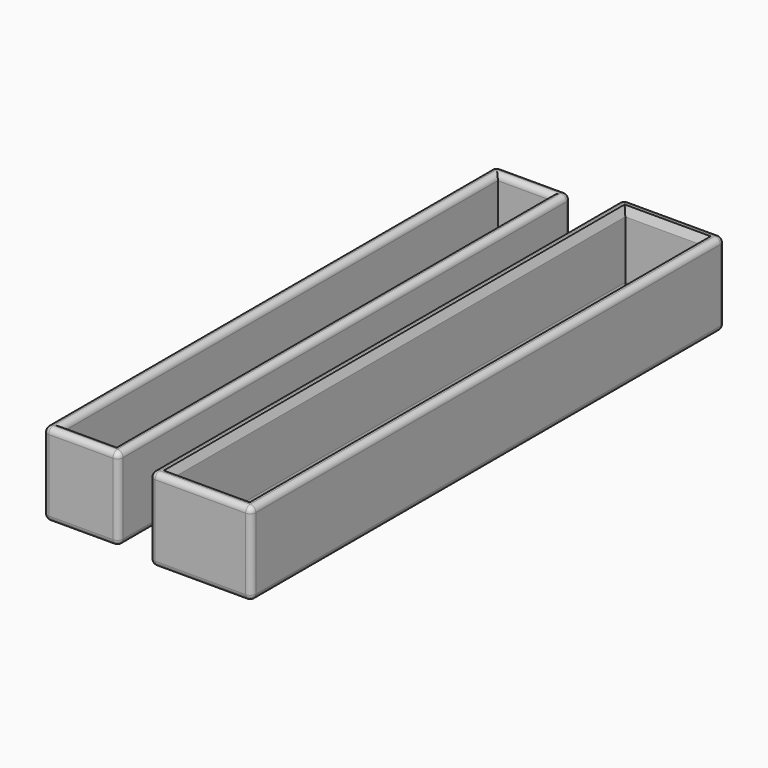
from build123d import *

# Parameters (mm, degrees)
F0_W          = 20
F0_H          = 150
F1_DEPTH      = 22
F2_T          = -3
F3_W          = 27
F3_H          = 157
F4_DEPTH      = 22
F5_T          = -3
F6_R          = 1.49999
F6_2_R        = 1.49999
F7_SIZE       = 0.9
F8_T4_DEPTH   = 21
F8_T9_DEPTH   = 24.3704715108
F8_T15_DEPTH  = 21
F8_T21_DEPTH  = 21
F8_T26_DEPTH  = 24.3704715108
F8_T32_DEPTH  = 151
F8_T37_DEPTH  = 154.3704715108
F8_T43_DEPTH  = 151
F8_T49_DEPTH  = 151
F8_T54_DEPTH  = 154.3704715108
F8_T60_DEPTH  = 151
F8_T65_DEPTH  = 154.3704715108
F8_T71_DEPTH  = 151
F8_T77_DEPTH  = 151
F8_T82_DEPTH  = 154.3704715108
F8_T88_DEPTH  = 21
F8_T93_DEPTH  = 24.3704715108
F8_T99_DEPTH  = 21
F8_T105_DEPTH = 21
F8_T110_DEPTH = 24.3704715108
F8_T117_DEPTH = 24.3704715108
F8_T122_DEPTH = 154.3704715108
F8_T130_DEPTH = 24.3704715108
F8_T135_DEPTH = 154.3704715108
F8_T143_DEPTH = 154.3704715108
F8_T148_DEPTH = 24.3704715108
F8_T156_DEPTH = 154.3704715108
F8_T161_DEPTH = 24.3704715108


# Not quite as in the source:
# - a fillet or chamfer that OpenCascade refuses, or shapes differently, is made with other operations: its cross-section is extruded or revolved along the edge and cut away or added
# - a fillet or chamfer is up to 0.001 mm smaller than in the source, because OpenCascade refuses the exact size


with BuildPart() as f1:
    # F0 (on Top) → F1 (new body)
    with BuildSketch(Plane.XY):
        with Locations((-29.877627335, 2.0745843649)):
            Rectangle(F0_W, F0_H)
    extrude(amount=F1_DEPTH)

    # F2
    f2_openings = [f1.faces().sort_by_distance(p)[0] for p in [
        (-29.877627, 2.074584, 22),
    ]]
    offset(amount=F2_T, openings=f2_openings)

    # F6 (radius 1.5 in the source; OpenCascade refuses exactly that, so slightly less here)
    f6_edges = [f1.edges().sort_by_distance(p)[0] for p in [
        (-19.877627, 2.074584, 22),
        (-22.877627, 2.074584, 22),
        (-29.877627, 77.074584, 22),
        (-29.877627, 74.074584, 22),
        (-39.877627, 2.074584, 22),
        (-36.877627, 2.074584, 22),
        (-29.877627, -69.925416, 22),
        (-29.877627, -72.925416, 22),
        (-39.877627, 2.074584, 0),
        (-39.877627, -72.925416, 11),
        (-29.877627, -72.925416, 0),
        (-19.877627, -72.925416, 11),
        (-19.877627, 77.074584, 11),
        (-39.877627, 77.074584, 11),
        (-29.877627, 77.074584, 0),
        (-19.877627, 2.074584, 0),
        (-36.877627, 2.074584, 3),
        (-29.877627, -69.925416, 3),
        (-29.877627, 74.074584, 3),
        (-22.877627, 2.074584, 3),
    ]]
    fillet(f6_edges, radius=F6_R)


with BuildPart() as f4:
    # F3 (on Top) → F4 (new body)
    with BuildSketch(Plane.XY):
        with Locations((3.5, 3.5)):
            Rectangle(F3_W, F3_H)
    extrude(amount=F4_DEPTH)

    # F5
    f5_openings = [f4.faces().sort_by_distance(p)[0] for p in [
        (3.5, 3.5, 22),
    ]]
    offset(amount=F5_T, openings=f5_openings)

    # F6#2 (radius 1.5 in the source; OpenCascade refuses exactly that, so slightly less here)
    f6_2_edges = [f4.edges().sort_by_distance(p)[0] for p in [
        (3.5, 82, 22),
        (-10, 3.5, 22),
        (17, 3.5, 22),
        (3.5, -75, 22),
        (3.5, -75, 0),
        (17, -75, 11),
        (17, 3.5, 0),
        (-10, 3.5, 0),
        (-10, -75, 11),
        (-10, 82, 11),
        (17, 82, 11),
        (3.5, 82, 0),
        (3.5, 79, 3),
        (14, 3.5, 3),
        (-7, 3.5, 3),
        (3.5, -72, 3),
    ]]
    fillet(f6_2_edges, radius=F6_2_R)

    # F7
    f7_edges = [f4.edges().sort_by_distance(p)[0] for p in [
        (3.5, 79, 22),
        (-7, 3.5, 22),
        (14, 3.5, 22),
        (3.5, -72, 22),
    ]]
    chamfer(f7_edges, length=F7_SIZE)

    # F8: chamfer of 1.3 on 4 edges, made by hand


with BuildPart() as f8_tool2:
    # F8_s3 → F8_t4 (new body)
    with BuildSketch(Plane.YZ.offset(14)):
        Polygon((79.9192388155, 22.0192388155), (79, 19.8), (79, 21.1), align=None)
    extrude(amount=-F8_T4_DEPTH)

    split(bisect_by=Plane(origin=(-3.55, 0, 3.55), x_dir=(0, 1, 0), z_dir=(0.7071067812, 0, -0.7071067812)), keep=Keep.TOP)


with BuildPart() as f4_1:
    add(f4.part)

    # F8_t1: cut F8_tool2
    add(f8_tool2.part, mode=Mode.SUBTRACT)


with BuildPart() as f8_tool7:
    # F8_s8 → F8_t9 (new body)
    with BuildSketch(Plane.YZ.offset(17.3704715108)):
        Polygon((79.9192388155, 22.0192388155), (79, 19.8), (79, 21.1), align=None)
    extrude(amount=-F8_T9_DEPTH)

    split(bisect_by=Plane(origin=(-3.55, 0, 3.55), x_dir=(0, 1, 0), z_dir=(-0.7071067812, 0, 0.7071067812)), keep=Keep.TOP)

    split(bisect_by=Plane.YZ.offset(14), keep=Keep.TOP)


with BuildPart() as f4_2:
    add(f4_1.part)

    # F8_t6: cut F8_tool7
    add(f8_tool7.part, mode=Mode.SUBTRACT)


with BuildPart() as f8_tool13:
    # F8_s14 → F8_t15 (new body)
    with BuildSketch(Plane.YZ.offset(14)):
        Polygon((79.9192388155, 22.0192388155), (79, 19.8), (79, 21.1), align=None)
    extrude(amount=-F8_T15_DEPTH)

    split(bisect_by=Plane(origin=(-3.55, 0, 3.55), x_dir=(0, 1, 0), z_dir=(-0.7071067812, 0, 0.7071067812)), keep=Keep.TOP)

    split(bisect_by=Plane(origin=(7.05, 0, 7.05), x_dir=(0, 1, 0), z_dir=(0.7071067812, 0, 0.7071067812)), keep=Keep.TOP)


with BuildPart() as f4_3:
    add(f4_2.part)

    # F8_t12: cut F8_tool13
    add(f8_tool13.part, mode=Mode.SUBTRACT)


with BuildPart() as f8_tool19:
    # F8_s20 → F8_t21 (new body)
    with BuildSketch(Plane.YZ.offset(14)):
        Polygon((79.9192388155, 22.0192388155), (79, 19.8), (79, 21.1), align=None)
    extrude(amount=-F8_T21_DEPTH)

    split(bisect_by=Plane(origin=(7.05, 0, 7.05), x_dir=(0, 1, 0), z_dir=(-0.7071067812, 0, -0.7071067812)), keep=Keep.TOP)


with BuildPart() as f4_4:
    add(f4_3.part)

    # F8_t18: cut F8_tool19
    add(f8_tool19.part, mode=Mode.SUBTRACT)


with BuildPart() as f8_tool24:
    # F8_s25 → F8_t26 (new body)
    with BuildSketch(Plane.YZ.offset(14)):
        Polygon((79.9192388155, 22.0192388155), (79, 19.8), (79, 21.1), align=None)
    extrude(amount=-F8_T26_DEPTH)

    split(bisect_by=Plane(origin=(7.05, 0, 7.05), x_dir=(0, 1, 0), z_dir=(0.7071067812, 0, 0.7071067812)), keep=Keep.TOP)

    split(bisect_by=Plane.YZ.offset(-7), keep=Keep.BOTTOM)


with BuildPart() as f4_5:
    add(f4_4.part)

    # F8_t23: cut F8_tool24
    add(f8_tool24.part, mode=Mode.SUBTRACT)


with BuildPart() as f8_tool30:
    # F8_s31 → F8_t32 (new body)
    with BuildSketch(Plane.XZ.offset(-79)):
        Polygon((-7.9192388155, 22.0192388155), (-7, 19.8), (-7, 21.1), align=None)
    extrude(amount=F8_T32_DEPTH)

    split(bisect_by=Plane(origin=(0, 28.95, -28.95), x_dir=(1, 0, 0), z_dir=(0, 0.7071067812, -0.7071067812)), keep=Keep.TOP)


with BuildPart() as f4_6:
    add(f4_5.part)

    # F8_t29: cut F8_tool30
    add(f8_tool30.part, mode=Mode.SUBTRACT)


with BuildPart() as f8_tool35:
    # F8_s36 → F8_t37 (new body)
    with BuildSketch(Plane.XZ.offset(-82.3704715108)):
        Polygon((-7.9192388155, 22.0192388155), (-7, 19.8), (-7, 21.1), align=None)
    extrude(amount=F8_T37_DEPTH)

    split(bisect_by=Plane(origin=(0, 28.95, -28.95), x_dir=(1, 0, 0), z_dir=(0, -0.7071067812, 0.7071067812)), keep=Keep.TOP)

    split(bisect_by=Plane.XZ.offset(-79), keep=Keep.BOTTOM)


with BuildPart() as f4_7:
    add(f4_6.part)

    # F8_t34: cut F8_tool35
    add(f8_tool35.part, mode=Mode.SUBTRACT)


with BuildPart() as f8_tool41:
    # F8_s42 → F8_t43 (new body)
    with BuildSketch(Plane.XZ.offset(-79)):
        Polygon((-7.9192388155, 22.0192388155), (-7, 19.8), (-7, 21.1), align=None)
    extrude(amount=F8_T43_DEPTH)

    split(bisect_by=Plane(origin=(0, 28.95, -28.95), x_dir=(1, 0, 0), z_dir=(0, -0.7071067812, 0.7071067812)), keep=Keep.TOP)

    split(bisect_by=Plane(origin=(0, -25.45, -25.45), x_dir=(1, 0, 0), z_dir=(0, 0.7071067812, 0.7071067812)), keep=Keep.TOP)


with BuildPart() as f4_8:
    add(f4_7.part)

    # F8_t40: cut F8_tool41
    add(f8_tool41.part, mode=Mode.SUBTRACT)


with BuildPart() as f8_tool47:
    # F8_s48 → F8_t49 (new body)
    with BuildSketch(Plane.XZ.offset(-79)):
        Polygon((-7.9192388155, 22.0192388155), (-7, 19.8), (-7, 21.1), align=None)
    extrude(amount=F8_T49_DEPTH)

    split(bisect_by=Plane(origin=(0, -25.45, -25.45), x_dir=(1, 0, 0), z_dir=(0, -0.7071067812, -0.7071067812)), keep=Keep.TOP)


with BuildPart() as f4_9:
    add(f4_8.part)

    # F8_t46: cut F8_tool47
    add(f8_tool47.part, mode=Mode.SUBTRACT)


with BuildPart() as f8_tool52:
    # F8_s53 → F8_t54 (new body)
    with BuildSketch(Plane.XZ.offset(-79)):
        Polygon((-7.9192388155, 22.0192388155), (-7, 19.8), (-7, 21.1), align=None)
    extrude(amount=F8_T54_DEPTH)

    split(bisect_by=Plane(origin=(0, -25.45, -25.45), x_dir=(1, 0, 0), z_dir=(0, 0.7071067812, 0.7071067812)), keep=Keep.TOP)

    split(bisect_by=Plane.XZ.offset(72), keep=Keep.TOP)


with BuildPart() as f4_10:
    add(f4_9.part)

    # F8_t51: cut F8_tool52
    add(f8_tool52.part, mode=Mode.SUBTRACT)


with BuildPart() as f8_tool58:
    # F8_s59 → F8_t60 (new body)
    with BuildSketch(Plane.XZ.offset(72)):
        Polygon((14.9192388155, 22.0192388155), (14, 19.8), (14, 21.1), align=None)
    extrude(amount=-F8_T60_DEPTH)

    split(bisect_by=Plane(origin=(0, -25.45, -25.45), x_dir=(1, 0, 0), z_dir=(0, -0.7071067812, -0.7071067812)), keep=Keep.TOP)


with BuildPart() as f4_11:
    add(f4_10.part)

    # F8_t57: cut F8_tool58
    add(f8_tool58.part, mode=Mode.SUBTRACT)


with BuildPart() as f8_tool63:
    # F8_s64 → F8_t65 (new body)
    with BuildSketch(Plane.XZ.offset(75.3704715108)):
        Polygon((14.9192388155, 22.0192388155), (14, 19.8), (14, 21.1), align=None)
    extrude(amount=-F8_T65_DEPTH)

    split(bisect_by=Plane(origin=(0, -25.45, -25.45), x_dir=(1, 0, 0), z_dir=(0, 0.7071067812, 0.7071067812)), keep=Keep.TOP)

    split(bisect_by=Plane.XZ.offset(72), keep=Keep.TOP)


with BuildPart() as f4_12:
    add(f4_11.part)

    # F8_t62: cut F8_tool63
    add(f8_tool63.part, mode=Mode.SUBTRACT)


with BuildPart() as f8_tool69:
    # F8_s70 → F8_t71 (new body)
    with BuildSketch(Plane.XZ.offset(72)):
        Polygon((14.9192388155, 22.0192388155), (14, 19.8), (14, 21.1), align=None)
    extrude(amount=-F8_T71_DEPTH)

    split(bisect_by=Plane(origin=(0, 28.95, -28.95), x_dir=(1, 0, 0), z_dir=(0, -0.7071067812, 0.7071067812)), keep=Keep.TOP)

    split(bisect_by=Plane(origin=(0, -25.45, -25.45), x_dir=(1, 0, 0), z_dir=(0, 0.7071067812, 0.7071067812)), keep=Keep.TOP)


with BuildPart() as f4_13:
    add(f4_12.part)

    # F8_t68: cut F8_tool69
    add(f8_tool69.part, mode=Mode.SUBTRACT)


with BuildPart() as f8_tool75:
    # F8_s76 → F8_t77 (new body)
    with BuildSketch(Plane.XZ.offset(72)):
        Polygon((14.9192388155, 22.0192388155), (14, 19.8), (14, 21.1), align=None)
    extrude(amount=-F8_T77_DEPTH)

    split(bisect_by=Plane(origin=(0, 28.95, -28.95), x_dir=(1, 0, 0), z_dir=(0, 0.7071067812, -0.7071067812)), keep=Keep.TOP)


with BuildPart() as f4_14:
    add(f4_13.part)

    # F8_t74: cut F8_tool75
    add(f8_tool75.part, mode=Mode.SUBTRACT)


with BuildPart() as f8_tool80:
    # F8_s81 → F8_t82 (new body)
    with BuildSketch(Plane.XZ.offset(72)):
        Polygon((14.9192388155, 22.0192388155), (14, 19.8), (14, 21.1), align=None)
    extrude(amount=-F8_T82_DEPTH)

    split(bisect_by=Plane(origin=(0, 28.95, -28.95), x_dir=(1, 0, 0), z_dir=(0, -0.7071067812, 0.7071067812)), keep=Keep.TOP)

    split(bisect_by=Plane.XZ.offset(-79), keep=Keep.BOTTOM)


with BuildPart() as f4_15:
    add(f4_14.part)

    # F8_t79: cut F8_tool80
    add(f8_tool80.part, mode=Mode.SUBTRACT)


with BuildPart() as f8_tool86:
    # F8_s87 → F8_t88 (new body)
    with BuildSketch(Plane.YZ.offset(-7)):
        Polygon((-72.9192388155, 22.0192388155), (-72, 19.8), (-72, 21.1), align=None)
    extrude(amount=F8_T88_DEPTH)

    split(bisect_by=Plane(origin=(7.05, 0, 7.05), x_dir=(0, 1, 0), z_dir=(-0.7071067812, 0, -0.7071067812)), keep=Keep.TOP)


with BuildPart() as f4_16:
    add(f4_15.part)

    # F8_t85: cut F8_tool86
    add(f8_tool86.part, mode=Mode.SUBTRACT)


with BuildPart() as f8_tool91:
    # F8_s92 → F8_t93 (new body)
    with BuildSketch(Plane.YZ.offset(-10.3704715108)):
        Polygon((-72.9192388155, 22.0192388155), (-72, 19.8), (-72, 21.1), align=None)
    extrude(amount=F8_T93_DEPTH)

    split(bisect_by=Plane(origin=(7.05, 0, 7.05), x_dir=(0, 1, 0), z_dir=(0.7071067812, 0, 0.7071067812)), keep=Keep.TOP)

    split(bisect_by=Plane.YZ.offset(-7), keep=Keep.BOTTOM)


with BuildPart() as f4_17:
    add(f4_16.part)

    # F8_t90: cut F8_tool91
    add(f8_tool91.part, mode=Mode.SUBTRACT)


with BuildPart() as f8_tool97:
    # F8_s98 → F8_t99 (new body)
    with BuildSketch(Plane.YZ.offset(-7)):
        Polygon((-72.9192388155, 22.0192388155), (-72, 19.8), (-72, 21.1), align=None)
    extrude(amount=F8_T99_DEPTH)

    split(bisect_by=Plane(origin=(-3.55, 0, 3.55), x_dir=(0, 1, 0), z_dir=(-0.7071067812, 0, 0.7071067812)), keep=Keep.TOP)

    split(bisect_by=Plane(origin=(7.05, 0, 7.05), x_dir=(0, 1, 0), z_dir=(0.7071067812, 0, 0.7071067812)), keep=Keep.TOP)


with BuildPart() as f4_18:
    add(f4_17.part)

    # F8_t96: cut F8_tool97
    add(f8_tool97.part, mode=Mode.SUBTRACT)


with BuildPart() as f8_tool103:
    # F8_s104 → F8_t105 (new body)
    with BuildSketch(Plane.YZ.offset(-7)):
        Polygon((-72.9192388155, 22.0192388155), (-72, 19.8), (-72, 21.1), align=None)
    extrude(amount=F8_T105_DEPTH)

    split(bisect_by=Plane(origin=(-3.55, 0, 3.55), x_dir=(0, 1, 0), z_dir=(0.7071067812, 0, -0.7071067812)), keep=Keep.TOP)


with BuildPart() as f4_19:
    add(f4_18.part)

    # F8_t102: cut F8_tool103
    add(f8_tool103.part, mode=Mode.SUBTRACT)


with BuildPart() as f8_tool108:
    # F8_s109 → F8_t110 (new body)
    with BuildSketch(Plane.YZ.offset(-7)):
        Polygon((-72.9192388155, 22.0192388155), (-72, 19.8), (-72, 21.1), align=None)
    extrude(amount=F8_T110_DEPTH)

    split(bisect_by=Plane(origin=(-3.55, 0, 3.55), x_dir=(0, 1, 0), z_dir=(-0.7071067812, 0, 0.7071067812)), keep=Keep.TOP)

    split(bisect_by=Plane.YZ.offset(14), keep=Keep.TOP)


with BuildPart() as f4_20:
    add(f4_19.part)

    # F8_t107: cut F8_tool108
    add(f8_tool108.part, mode=Mode.SUBTRACT)


with BuildPart() as f8_tool115:
    # F8_s116 → F8_t117 (new body)
    with BuildSketch(Plane.YZ.offset(17.3704715108)):
        Polygon((79.9192388155, 22.0192388155), (79, 19.8), (79, 21.1), align=None)
    extrude(amount=-F8_T117_DEPTH)

    split(bisect_by=Plane(origin=(-3.55, 0, 3.55), x_dir=(0, 1, 0), z_dir=(0.7071067812, 0, -0.7071067812)), keep=Keep.TOP)

    split(bisect_by=Plane.YZ.offset(14), keep=Keep.TOP)


with BuildPart() as f8_tool120:
    # F8_s121 → F8_t122 (new body)
    with BuildSketch(Plane.XZ.offset(72)):
        Polygon((14.9192388155, 22.0192388155), (14, 19.8), (14, 21.1), align=None)
    extrude(amount=-F8_T122_DEPTH)

    split(bisect_by=Plane(origin=(0, 28.95, -28.95), x_dir=(1, 0, 0), z_dir=(0, 0.7071067812, -0.7071067812)), keep=Keep.TOP)

    split(bisect_by=Plane.XZ.offset(-79), keep=Keep.BOTTOM)


with BuildPart() as f8_tool115_1:
    add(f8_tool115.part)

    # F8_t125: intersect F8_tool120
    add(f8_tool120.part, mode=Mode.INTERSECT)


with BuildPart() as f4_21:
    add(f4_20.part)

    # F8_t113: cut F8_tool115
    add(f8_tool115_1.part, mode=Mode.SUBTRACT)


with BuildPart() as f8_tool128:
    # F8_s129 → F8_t130 (new body)
    with BuildSketch(Plane.YZ.offset(14)):
        Polygon((79.9192388155, 22.0192388155), (79, 19.8), (79, 21.1), align=None)
    extrude(amount=-F8_T130_DEPTH)

    split(bisect_by=Plane(origin=(7.05, 0, 7.05), x_dir=(0, 1, 0), z_dir=(-0.7071067812, 0, -0.7071067812)), keep=Keep.TOP)

    split(bisect_by=Plane.YZ.offset(-7), keep=Keep.BOTTOM)


with BuildPart() as f8_tool133:
    # F8_s134 → F8_t135 (new body)
    with BuildSketch(Plane.XZ.offset(-82.3704715108)):
        Polygon((-7.9192388155, 22.0192388155), (-7, 19.8), (-7, 21.1), align=None)
    extrude(amount=F8_T135_DEPTH)

    split(bisect_by=Plane(origin=(0, 28.95, -28.95), x_dir=(1, 0, 0), z_dir=(0, 0.7071067812, -0.7071067812)), keep=Keep.TOP)

    split(bisect_by=Plane.XZ.offset(-79), keep=Keep.BOTTOM)


with BuildPart() as f8_tool128_1:
    add(f8_tool128.part)

    # F8_t138: intersect F8_tool133
    add(f8_tool133.part, mode=Mode.INTERSECT)


with BuildPart() as f4_22:
    add(f4_21.part)

    # F8_t126: cut F8_tool128
    add(f8_tool128_1.part, mode=Mode.SUBTRACT)


with BuildPart() as f8_tool141:
    # F8_s142 → F8_t143 (new body)
    with BuildSketch(Plane.XZ.offset(-79)):
        Polygon((-7.9192388155, 22.0192388155), (-7, 19.8), (-7, 21.1), align=None)
    extrude(amount=F8_T143_DEPTH)

    split(bisect_by=Plane(origin=(0, -25.45, -25.45), x_dir=(1, 0, 0), z_dir=(0, -0.7071067812, -0.7071067812)), keep=Keep.TOP)

    split(bisect_by=Plane.XZ.offset(72), keep=Keep.TOP)


with BuildPart() as f8_tool146:
    # F8_s147 → F8_t148 (new body)
    with BuildSketch(Plane.YZ.offset(-10.3704715108)):
        Polygon((-72.9192388155, 22.0192388155), (-72, 19.8), (-72, 21.1), align=None)
    extrude(amount=F8_T148_DEPTH)

    split(bisect_by=Plane(origin=(7.05, 0, 7.05), x_dir=(0, 1, 0), z_dir=(-0.7071067812, 0, -0.7071067812)), keep=Keep.TOP)

    split(bisect_by=Plane.YZ.offset(-7), keep=Keep.BOTTOM)


with BuildPart() as f8_tool141_1:
    add(f8_tool141.part)

    # F8_t151: intersect F8_tool146
    add(f8_tool146.part, mode=Mode.INTERSECT)


with BuildPart() as f4_23:
    add(f4_22.part)

    # F8_t139: cut F8_tool141
    add(f8_tool141_1.part, mode=Mode.SUBTRACT)


with BuildPart() as f8_tool154:
    # F8_s155 → F8_t156 (new body)
    with BuildSketch(Plane.XZ.offset(75.3704715108)):
        Polygon((14.9192388155, 22.0192388155), (14, 19.8), (14, 21.1), align=None)
    extrude(amount=-F8_T156_DEPTH)

    split(bisect_by=Plane(origin=(0, -25.45, -25.45), x_dir=(1, 0, 0), z_dir=(0, -0.7071067812, -0.7071067812)), keep=Keep.TOP)

    split(bisect_by=Plane.XZ.offset(72), keep=Keep.TOP)


with BuildPart() as f8_tool159:
    # F8_s160 → F8_t161 (new body)
    with BuildSketch(Plane.YZ.offset(-7)):
        Polygon((-72.9192388155, 22.0192388155), (-72, 19.8), (-72, 21.1), align=None)
    extrude(amount=F8_T161_DEPTH)

    split(bisect_by=Plane(origin=(-3.55, 0, 3.55), x_dir=(0, 1, 0), z_dir=(0.7071067812, 0, -0.7071067812)), keep=Keep.TOP)

    split(bisect_by=Plane.YZ.offset(14), keep=Keep.TOP)


with BuildPart() as f8_tool154_1:
    add(f8_tool154.part)

    # F8_t164: intersect F8_tool159
    add(f8_tool159.part, mode=Mode.INTERSECT)


with BuildPart() as f4_24:
    add(f4_23.part)

    # F8_t152: cut F8_tool154
    add(f8_tool154_1.part, mode=Mode.SUBTRACT)


solid = Compound([f1.part, f4_24.part])
